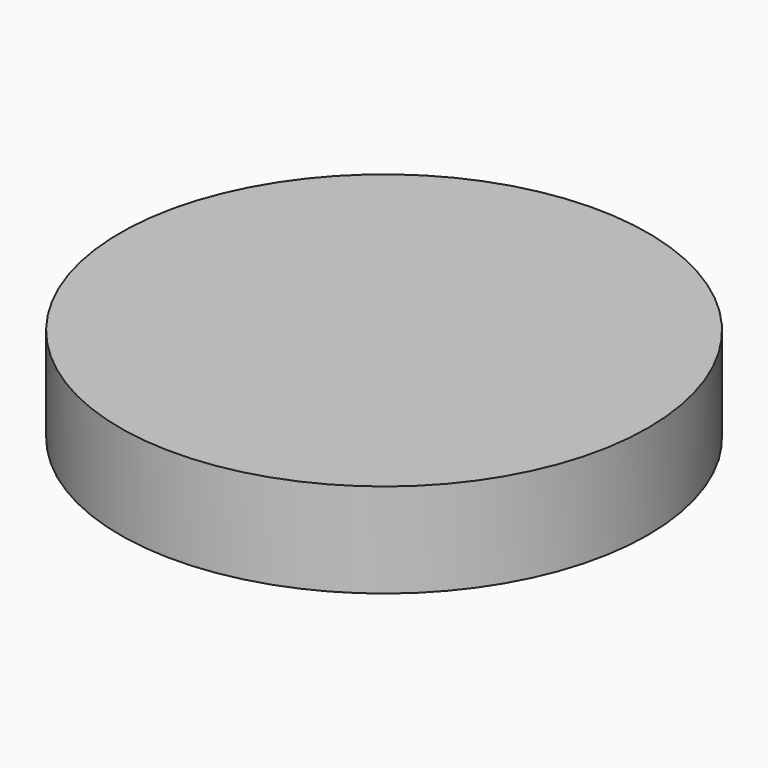
from build123d import *

# Parameters (mm, degrees)
F2_R     = 28
F3_DEPTH = 10


# Not quite as in the source:
# - the program builds the solid bodies; features that only make, move or delete a surface that nothing else refers to are left out


with BuildPart() as f3:
    # F2 (on Top) → F3 (new body)
    with BuildSketch(Plane.XY):
        with Locations((-46.3043488562, 17.1195659786)):
            Circle(F2_R)
    extrude(amount=F3_DEPTH)


solid = f3.part
